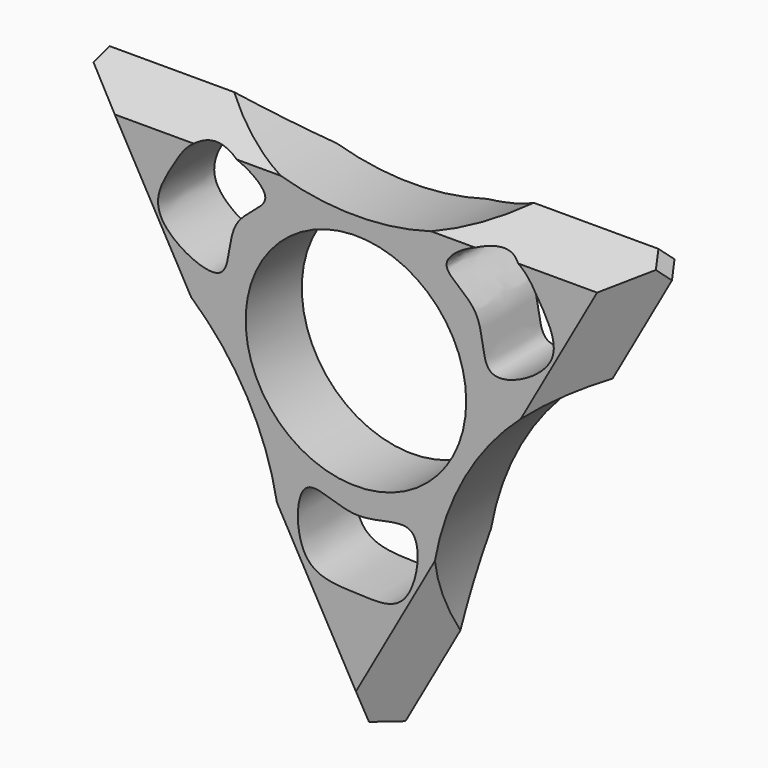
from build123d import *

# Parameters (mm, degrees)
F0_R         = 11
F1_DEPTH     = 7
F2_T1_DEPTH  = 35.2813832436
F2_T3_DEPTH  = 35.5467430765
F2_T5_DEPTH  = 34.4305362998
F2_T7_DEPTH  = 34.4305362998
F2_T9_DEPTH  = 35.2813832436
F2_T11_DEPTH = 35.5467430765


# Not quite as in the source:
# - a fillet or chamfer that OpenCascade refuses, or shapes differently, is made with other operations: its cross-section is extruded or revolved along the edge and cut away or added


with BuildPart() as f1:
    # F0 (on Front) → F1 (new body)
    with BuildSketch(Plane.XZ):
        with BuildLine():
            Line((-8.017778225, -25.1282889185), (-3.9536927291, -32.3677882552))
            Line((-3.9536927291, -32.3677882552), (3.9536927291, -32.3677882552))
            Line((3.9536927291, -32.3677882552), (8.017778225, -25.1282889185))
            ThreePointArc((8.017778225, -25.1282889185), (10.8745416094, -6.6499044579), (25.1621004057, 5.4114989824))
            Line((25.1621004057, 5.4114989824), (29.6426898708, 13.3929315811))
            Line((29.6426898708, 13.3929315811), (26.4639375252, 18.8986921484))
            Line((26.4639375252, 18.8986921484), (17.0454936065, 18.8986921484))
            ThreePointArc((17.0454936065, 18.8986921484), (0, 12.7406410493), (-17.0454936065, 18.8986921484))
            Line((-17.0454936065, 18.8986921484), (-26.4639375252, 18.8986921484))
            Line((-26.4639375252, 18.8986921484), (-29.6426898708, 13.3929315811))
            Line((-29.6426898708, 13.3929315811), (-25.1621004057, 5.4114989824))
            ThreePointArc((-25.1621004057, 5.4114989824), (-12.3306252771, -4.3414248541), (-7.4606163281, -19.7053205246))
            ThreePointArc((-7.4606163281, -19.7053205246), (-7.6002724535, -22.4310780148), (-8.017778225, -25.1282889185))
        make_face()
        Circle(F0_R, mode=Mode.SUBTRACT)
        with BuildLine():
            add(Edge.make_bspline(
                [(-19.3735472858, 6.192852743), (-18.3495240804, 4.3809635142), (-11.9151294961, 1.0595732713), (-13.3041344414, 8.8422203653), (-6.4288769454, 11.2946801857), (-15.4136761166, 16.0382229659), (-18.410160006, 11.0468887375), (-20.2663386903, 7.7725426571), (-19.3735472858, 6.192852743)],
                knots=[0, 0, 0, 0, 0.1830546722, 0.3457253498, 0.4974713646, 0.6774626151, 0.8404043609, 1, 1, 1, 1], degree=3))
        make_face(mode=Mode.SUBTRACT)
        with BuildLine():
            add(Edge.make_bspline(
                [(-4.9653253518, -12.7779729664), (-3.9673538813, -11.990438984), (-0.0815721197, -14.8647438543), (7.1063785889, -10.9230753891), (5.7028649477, -20.847724526), (0.130602412, -20.2827447937), (-6.1063753916, -20.3844092682), (-6.0569718905, -13.6394292017), (-4.9653253518, -12.7779729664)],
                knots=[0, 0, 0, 0, 0.1595531099, 0.3282047144, 0.5033592864, 0.6613074183, 0.8254703614, 1, 1, 1, 1], degree=3))
        make_face(mode=Mode.SUBTRACT)
        with BuildLine():
            add(Edge.make_bspline(
                [(19.3735472858, 6.192852743), (18.3495240804, 4.3809635142), (11.9151294961, 1.0595732713), (13.3041344414, 8.8422203653), (6.4288769454, 11.2946801857), (15.4136761166, 16.0382229659), (18.410160006, 11.0468887375), (20.2663386903, 7.7725426571), (19.3735472858, 6.192852743)],
                knots=[0, 0, 0, 0, 0.1830546722, 0.3457253498, 0.4974713646, 0.6774626151, 0.8404043609, 1, 1, 1, 1], degree=3))
        make_face(mode=Mode.SUBTRACT)
    extrude(amount=F1_DEPTH)

    # F2: chamfer of 5.08 on 12 edges, made by hand

    # F2_s2 → F2_t1 (cut)
    with BuildSketch(Plane(origin=(-19.2151547034, 0, 34.2286351679), x_dir=(0, 1, 0), z_dir=(0.4895169129, 0, -0.8719938027))):
        Polygon((-7, -14.2121753414), (-1.92, -19.2921753414), (-7, -19.2921753414), align=None)
        Polygon((-5.08, -19.2921753414), (0, -14.2121753414), (0, -19.2921753414), align=None)
    extrude(amount=F2_T1_DEPTH, mode=Mode.SUBTRACT)

    # F2_s4 → F2_t3 (cut)
    with BuildSketch(Plane.YZ.offset(-39.5280871041)):
        Polygon((-7, 13.8186921484), (-1.92, 18.8986921484), (-7, 18.8986921484), align=None)
        Polygon((-5.08, 18.8986921484), (0, 13.8186921484), (0, 18.8986921484), align=None)
    extrude(amount=F2_T3_DEPTH, mode=Mode.SUBTRACT)

    # F2_s6 → F2_t5 (cut)
    with BuildSketch(Plane(origin=(-19.2640867811, 0, -34.3157996098), x_dir=(0, 1, 0), z_dir=(0.4895169129, 0, 0.8719938027))):
        Polygon((-7, -14.2121753414), (-1.92, -19.2921753414), (-7, -19.2921753414), align=None)
        Polygon((-5.08, -19.2921753414), (0, -14.2121753414), (0, -19.2921753414), align=None)
    extrude(amount=F2_T5_DEPTH, mode=Mode.SUBTRACT)

    # F2_s8 → F2_t7 (cut)
    with BuildSketch(Plane(origin=(2.4097569425, 0, -4.2925853318), x_dir=(0, 1, 0), z_dir=(0.4895169129, 0, -0.8719938027))):
        Polygon((-1.92, -19.2921753414), (-7, -14.2121753414), (-7, -19.2921753414), align=None)
        Polygon((-5.08, -19.2921753414), (0, -14.2121753414), (0, -19.2921753414), align=None)
    extrude(amount=F2_T7_DEPTH, mode=Mode.SUBTRACT)

    # F2_s10 → F2_t9 (cut)
    with BuildSketch(Plane(origin=(1.9443208955, 0, 3.4634876278), x_dir=(0, 1, 0), z_dir=(0.4895169129, 0, 0.8719938027))):
        Polygon((-7, -14.2121753414), (-1.92, -19.2921753414), (-7, -19.2921753414), align=None)
        Polygon((-5.08, -19.2921753414), (0, -14.2121753414), (0, -19.2921753414), align=None)
    extrude(amount=F2_T9_DEPTH, mode=Mode.SUBTRACT)

    # F2_s12 → F2_t11 (cut)
    with BuildSketch(Plane.YZ.offset(3.9813440276)):
        Polygon((-7, 13.8186921484), (-1.92, 18.8986921484), (-7, 18.8986921484), align=None)
        Polygon((-5.08, 18.8986921484), (0, 13.8186921484), (0, 18.8986921484), align=None)
    extrude(amount=F2_T11_DEPTH, mode=Mode.SUBTRACT)


solid = f1.part
